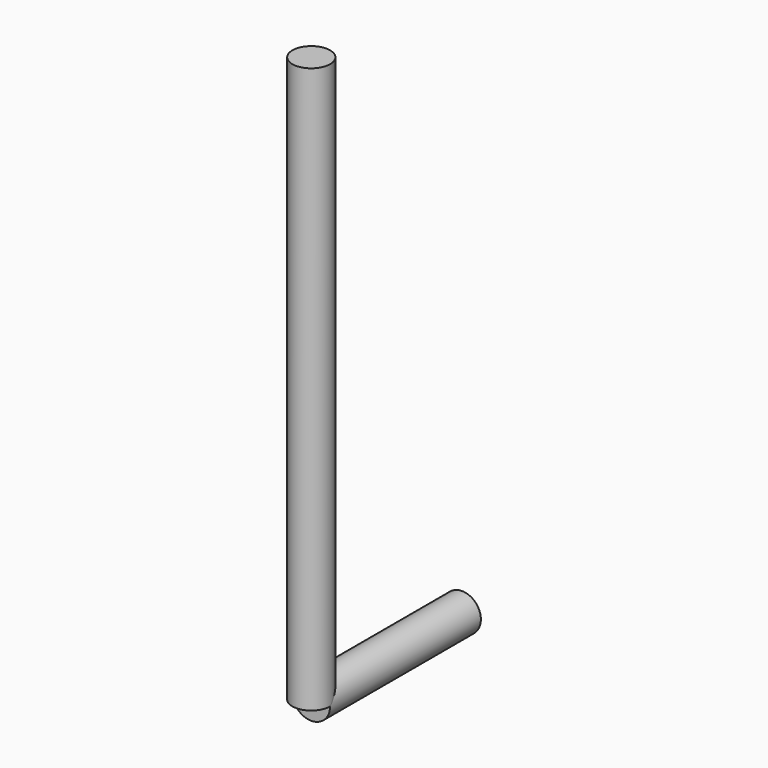
from build123d import *

# Parameters (mm, degrees)
F0_R     = 25.4
F1_DEPTH = 762
F4_R     = 25.4
F5_DEPTH = 254


# Not quite as in the source:
# - the program builds the solid bodies; features that only make, move or delete a surface that nothing else refers to are left out


with BuildPart() as f1:
    # F0 (on Top) → F1 (new body)
    with BuildSketch(Plane.XY):
        Circle(F0_R)
    extrude(amount=F1_DEPTH)

    # F4 (on Front) → F5 (join)
    with BuildSketch(Plane.XZ):
        Circle(F4_R)
    extrude(amount=-F5_DEPTH)


solid = f1.part
